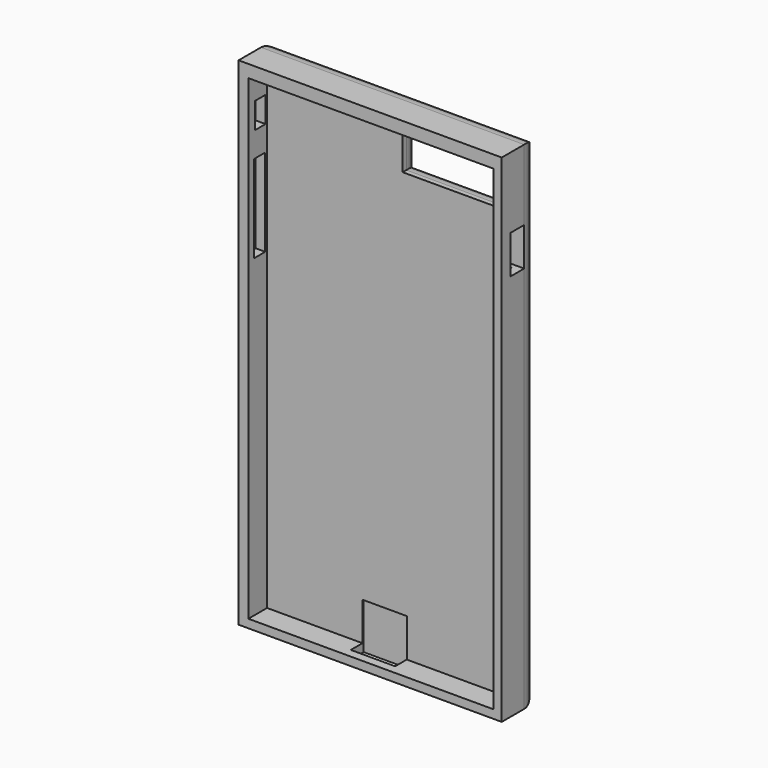
from build123d import *

# Parameters (mm, degrees)
F0_W          = 71.5089328587
F0_H          = 135.0168734789
F1_DEPTH      = 12.7
F2_W          = 66.5551535785
F2_H          = 129.3334215879
F3_DEPTH      = 3.175
F4_W          = 29.7537194565
F4_H          = 13.0016170442
F5_DEPTH      = 12.7
F6_T1_DEPTH   = 96.9089328587
F6_T3_DEPTH   = 160.4168734789
F6_T5_DEPTH   = 13.0016170442
F6_T7_DEPTH   = 29.7537194565
F6_T13_DEPTH  = 25.7016170442
F6_T17_DEPTH  = 42.4537194565
F6_T24_DEPTH  = 25.7016170442
F6_T29_DEPTH  = 42.4537194565
F6_T37_DEPTH  = 42.4537194565
F6_T42_DEPTH  = 25.7016170442
F6_T50_DEPTH  = 25.7016170442
F6_T56_DEPTH  = 42.4537194565
F8_W          = 12.041549664
F8_H          = 4.3452125974
F9_DEPTH      = 12.7
F10_DEPTH     = 3.175
F11_W         = 4.6954765302
F11_H         = 10.42952016
F12_DEPTH     = 1.5875
F13_DEPTH     = 3.175
F14_DEPTH     = 3.175
F15_W         = 3.5004382953
F15_H         = 7.000874728
F16_DEPTH     = 6.35
F17_W         = 3.7472322583
F17_H         = 23.7555298954
F18_DEPTH     = 6.35
F19_TEXT_SIZE = 6.2507784201
F20_DEPTH     = 5.842
F21_TEXT_SIZE = 8.6816441682
F22_DEPTH     = 5.08


# Not quite as in the source:
# - a fillet or chamfer that OpenCascade refuses, or shapes differently, is made with other operations: its cross-section is extruded or revolved along the edge and cut away or added
# - Text() gives the source's letters only with a copy of the font that has no kerning and outlines rounded to 1/6400 em; it was checked with that copy


with BuildPart() as f1:
    # F0 (on Front) → F1 (new body)
    with BuildSketch(Plane.XZ):
        with Locations((-0.6250794977, -1.1251419783)):
            Rectangle(F0_W, F0_H)
    extrude(amount=F1_DEPTH)

    # F2 (on face) → F3 (cut)
    with BuildSketch(Plane.XZ.offset(12.7)):
        with Locations((-0.4404280335, -1.6757398844)):
            Rectangle(F2_W, F2_H)
    extrude(amount=-F3_DEPTH, mode=Mode.SUBTRACT)

    # F4 (on face) → F5 (cut)
    with BuildSketch(Plane(origin=(0, 0, 0), x_dir=(-1, 0, 0), z_dir=(0, 1, 0))):
        with Locations((-18.0022506975, 56.3820470124)):
            Rectangle(F4_W, F4_H)
    extrude(amount=-F5_DEPTH, mode=Mode.SUBTRACT)

    # F6: fillet of radius 5.08 on 8 edges, made by hand

    # F6_s2 → F6_t1 (cut)
    with BuildSketch(Plane.YZ.offset(-49.079545927)):
        with BuildLine():
            ThreePointArc((-5.08, 66.3832947612), (-1.4878975516, 64.8953972096), (0, 61.3032947612))
            Line((0, 61.3032947612), (0, 66.3832947612))
            Line((0, 66.3832947612), (-5.08, 66.3832947612))
        make_face()
        with BuildLine():
            ThreePointArc((0, -63.5535787177), (-1.4878975516, -67.1456811661), (-5.08, -68.6335787177))
            Line((-5.08, -68.6335787177), (0, -68.6335787177))
            Line((0, -68.6335787177), (0, -63.5535787177))
        make_face()
    extrude(amount=F6_T1_DEPTH, mode=Mode.SUBTRACT)

    # F6_s4 → F6_t3 (cut)
    with BuildSketch(Plane.XY.offset(-81.3335787177)):
        with BuildLine():
            ThreePointArc((35.1293869317, -5.08), (33.6414893801, -1.4878975516), (30.0493869317, 0))
            Line((30.0493869317, 0), (35.1293869317, 0))
            Line((35.1293869317, 0), (35.1293869317, -5.08))
        make_face()
        with BuildLine():
            ThreePointArc((-36.379545927, -5.08), (-34.8916483755, -1.4878975516), (-31.299545927, 0))
            Line((-31.299545927, 0), (-36.379545927, 0))
            Line((-36.379545927, 0), (-36.379545927, -5.08))
        make_face()
    extrude(amount=F6_T3_DEPTH, mode=Mode.SUBTRACT)

    # F6_s6 → F6_t5 (cut)
    with BuildSketch(Plane.XY.offset(49.8812384903)):
        with BuildLine():
            ThreePointArc((-1.9546090308, 0), (1.6374934176, -1.4878975516), (3.1253909692, -5.08))
            Line((3.1253909692, -5.08), (3.1253909692, 0))
            Line((3.1253909692, 0), (-1.9546090308, 0))
        make_face()
        with BuildLine():
            ThreePointArc((37.9591104257, 0), (34.3670079773, -1.4878975516), (32.8791104257, -5.08))
            Line((32.8791104257, -5.08), (32.8791104257, 0))
            Line((32.8791104257, 0), (37.9591104257, 0))
        make_face()
    extrude(amount=F6_T5_DEPTH, mode=Mode.SUBTRACT)

    # F6_s8 → F6_t7 (cut)
    with BuildSketch(Plane.YZ.offset(3.1253909692)):
        with BuildLine():
            ThreePointArc((0, 44.8012384903), (-1.4878975516, 48.3933409388), (-5.08, 49.8812384903))
            Line((-5.08, 49.8812384903), (0, 49.8812384903))
            Line((0, 49.8812384903), (0, 44.8012384903))
        make_face()
        with BuildLine():
            ThreePointArc((0, 67.9628555346), (-1.4878975516, 64.3707530861), (-5.08, 62.8828555346))
            Line((-5.08, 62.8828555346), (0, 62.8828555346))
            Line((0, 62.8828555346), (0, 67.9628555346))
        make_face()
    extrude(amount=F6_T7_DEPTH, mode=Mode.SUBTRACT)


with BuildPart() as f6_tool11:
    # F6_s12 → F6_t13 (new body)
    with BuildSketch(Plane.XY.offset(37.1812384903)):
        with BuildLine():
            ThreePointArc((-1.9546090308, 0), (1.6374934176, -1.4878975516), (3.1253909692, -5.08))
            Line((3.1253909692, -5.08), (3.1253909692, 0))
            Line((3.1253909692, 0), (-1.9546090308, 0))
        make_face()
    extrude(amount=F6_T13_DEPTH)

    split(bisect_by=Plane.XY.offset(49.8812384903), keep=Keep.BOTTOM)


with BuildPart() as f6_tool15:
    # F6_s16 → F6_t17 (new body)
    with BuildSketch(Plane.YZ.offset(32.8791104257)):
        with BuildLine():
            ThreePointArc((0, 44.8012384903), (-1.4878975516, 48.3933409388), (-5.08, 49.8812384903))
            Line((-5.08, 49.8812384903), (0, 49.8812384903))
            Line((0, 49.8812384903), (0, 44.8012384903))
        make_face()
    extrude(amount=-F6_T17_DEPTH)

    split(bisect_by=Plane.YZ.offset(3.1253909692), keep=Keep.BOTTOM)


with BuildPart() as f6_tool11_1:
    add(f6_tool11.part)

    # F6_t19: intersect F6_tool15
    add(f6_tool15.part, mode=Mode.INTERSECT)


with BuildPart() as f1_1:
    add(f1.part)

    # F6_t9: cut F6_tool11
    add(f6_tool11_1.part, mode=Mode.SUBTRACT)


with BuildPart() as f6_tool22:
    # F6_s23 → F6_t24 (new body)
    with BuildSketch(Plane.XY.offset(49.8812384903)):
        with BuildLine():
            ThreePointArc((-1.9546090308, 0), (1.6374934176, -1.4878975516), (3.1253909692, -5.08))
            Line((3.1253909692, -5.08), (3.1253909692, 0))
            Line((3.1253909692, 0), (-1.9546090308, 0))
        make_face()
    extrude(amount=F6_T24_DEPTH)

    split(bisect_by=Plane.XY.offset(66.3832947612), keep=Keep.BOTTOM)

    split(bisect_by=Plane.XY.offset(62.8828555346), keep=Keep.TOP)


with BuildPart() as f6_tool27:
    # F6_s28 → F6_t29 (new body)
    with BuildSketch(Plane.YZ.offset(-9.5746090308)):
        with BuildLine():
            ThreePointArc((0, 67.9628555346), (-1.4878975516, 64.3707530861), (-5.08, 62.8828555346))
            Line((-5.08, 62.8828555346), (0, 62.8828555346))
            Line((0, 62.8828555346), (0, 67.9628555346))
        make_face()
    extrude(amount=F6_T29_DEPTH)

    split(bisect_by=Plane.XY.offset(66.3832947612), keep=Keep.BOTTOM)

    split(bisect_by=Plane.YZ.offset(3.1253909692), keep=Keep.BOTTOM)


with BuildPart() as f6_tool22_1:
    add(f6_tool22.part)

    # F6_t32: intersect F6_tool27
    add(f6_tool27.part, mode=Mode.INTERSECT)


with BuildPart() as f1_2:
    add(f1_1.part)

    # F6_t20: cut F6_tool22
    add(f6_tool22_1.part, mode=Mode.SUBTRACT)


with BuildPart() as f6_tool35:
    # F6_s36 → F6_t37 (new body)
    with BuildSketch(Plane.YZ.offset(45.5791104257)):
        with BuildLine():
            ThreePointArc((0, 44.8012384903), (-1.4878975516, 48.3933409388), (-5.08, 49.8812384903))
            Line((-5.08, 49.8812384903), (0, 49.8812384903))
            Line((0, 49.8812384903), (0, 44.8012384903))
        make_face()
    extrude(amount=-F6_T37_DEPTH)

    split(bisect_by=Plane.YZ.offset(35.1293869317), keep=Keep.BOTTOM)

    split(bisect_by=Plane.YZ.offset(32.8791104257), keep=Keep.TOP)


with BuildPart() as f6_tool40:
    # F6_s41 → F6_t42 (new body)
    with BuildSketch(Plane.XY.offset(62.8828555346)):
        with BuildLine():
            ThreePointArc((37.9591104257, 0), (34.3670079773, -1.4878975516), (32.8791104257, -5.08))
            Line((32.8791104257, -5.08), (32.8791104257, 0))
            Line((32.8791104257, 0), (37.9591104257, 0))
        make_face()
    extrude(amount=-F6_T42_DEPTH)

    split(bisect_by=Plane.YZ.offset(35.1293869317), keep=Keep.BOTTOM)

    split(bisect_by=Plane.XY.offset(49.8812384903), keep=Keep.BOTTOM)


with BuildPart() as f6_tool35_1:
    add(f6_tool35.part)

    # F6_t45: intersect F6_tool40
    add(f6_tool40.part, mode=Mode.INTERSECT)


with BuildPart() as f1_3:
    add(f1_2.part)

    # F6_t33: cut F6_tool35
    add(f6_tool35_1.part, mode=Mode.SUBTRACT)


with BuildPart() as f6_tool48:
    # F6_s49 → F6_t50 (new body)
    with BuildSketch(Plane.XY.offset(75.5828555346)):
        with BuildLine():
            ThreePointArc((37.9591104257, 0), (34.3670079773, -1.4878975516), (32.8791104257, -5.08))
            Line((32.8791104257, -5.08), (32.8791104257, 0))
            Line((32.8791104257, 0), (37.9591104257, 0))
        make_face()
    extrude(amount=-F6_T50_DEPTH)

    split(bisect_by=Plane.XY.offset(66.3832947612), keep=Keep.BOTTOM)

    split(bisect_by=Plane.YZ.offset(35.1293869317), keep=Keep.BOTTOM)

    split(bisect_by=Plane.XY.offset(62.8828555346), keep=Keep.TOP)


with BuildPart() as f6_tool54:
    # F6_s55 → F6_t56 (new body)
    with BuildSketch(Plane.YZ.offset(3.1253909692)):
        with BuildLine():
            ThreePointArc((0, 67.9628555346), (-1.4878975516, 64.3707530861), (-5.08, 62.8828555346))
            Line((-5.08, 62.8828555346), (0, 62.8828555346))
            Line((0, 62.8828555346), (0, 67.9628555346))
        make_face()
    extrude(amount=F6_T56_DEPTH)

    split(bisect_by=Plane.XY.offset(66.3832947612), keep=Keep.BOTTOM)

    split(bisect_by=Plane.YZ.offset(35.1293869317), keep=Keep.BOTTOM)

    split(bisect_by=Plane.YZ.offset(32.8791104257), keep=Keep.TOP)


with BuildPart() as f6_tool48_1:
    add(f6_tool48.part)

    # F6_t60: intersect F6_tool54
    add(f6_tool54.part, mode=Mode.INTERSECT)


with BuildPart() as f1_4:
    add(f1_3.part)

    # F6_t46: cut F6_tool48
    add(f6_tool48_1.part, mode=Mode.SUBTRACT)

    # F8 (on face) → F9 (cut)
    with BuildSketch(Plane(origin=(0, 0, -68.6335787177), x_dir=(1, 0, 0), z_dir=(0, 0, -1))):
        with Locations((-1.775913639, 8.129889844)):
            Rectangle(F8_W, F8_H)
    extrude(amount=-F9_DEPTH, mode=Mode.SUBTRACT)

    # F10 (cut): a face of the model
    f10_faces = [f1_4.faces().sort_by_distance(p)[0] for p in [
        (-1.2987269052, -9.525, -3.5253605956),
    ]]
    extrude(f10_faces, amount=-F10_DEPTH, mode=Mode.SUBTRACT)

    # F11 (on face) → F12 (join)
    with BuildSketch(Plane.YZ.offset(35.1293869317)):
        with Locations((-7.4277382651, 41.9391449541)):
            Rectangle(F11_W, F11_H)
    extrude(amount=F12_DEPTH)

    # F13 (cut): a face of the model
    f13_faces = [f1_4.faces().sort_by_distance(p)[0] for p in [
        (36.7168869317, -7.4277382651, 41.9391449541),
    ]]
    extrude(f13_faces, amount=-F13_DEPTH, mode=Mode.SUBTRACT)

    # F14 (cut): a face of the model
    f14_faces = [f1_4.faces().sort_by_distance(p)[0] for p in [
        (33.5418869317, -7.4277382651, 41.9391449541),
    ]]
    extrude(f14_faces, amount=-F14_DEPTH, mode=Mode.SUBTRACT)

    # F15 (on face) → F16 (cut)
    with BuildSketch(Plane(origin=(-36.379545927, 0, 0), x_dir=(0, -1, 0), z_dir=(-1, 0, 0))):
        with Locations((8.6260777898, 53.1316418201)):
            Rectangle(F15_W, F15_H)
    extrude(amount=-F16_DEPTH, mode=Mode.SUBTRACT)

    # F17 (on face) → F18 (cut)
    with BuildSketch(Plane(origin=(-36.379545927, 0, 0), x_dir=(0, -1, 0), z_dir=(-1, 0, 0))):
        with Locations((8.8518634439, 30.9905847535)):
            Rectangle(F17_W, F17_H)
    extrude(amount=-F18_DEPTH, mode=Mode.SUBTRACT)

    # F19 (on face) → F20 (join)
    with BuildSketch(Plane(origin=(0, 0, 0), x_dir=(-1, 0, 0), z_dir=(0, 1, 0))):
        with Locations((-18.8773591071, -49.6261417866)):
            Text('Palm Tree', F19_TEXT_SIZE, font='Open Sans', text_align=(TextAlign.LEFT, TextAlign.BOTTOM))
        with Locations((-18.8773591071, -58.1272004379)):
            Text('Phone Cases', F19_TEXT_SIZE, font='Open Sans', text_align=(TextAlign.LEFT, TextAlign.BOTTOM))
    extrude(amount=-F20_DEPTH)

    # F21 (on face) → F22 (cut)
    with BuildSketch(Plane(origin=(0, 0, 0), x_dir=(-1, 0, 0), z_dir=(0, 1, 0))):
        with Locations((-24.3780473247, -44.6305759251)):
            Text('Palm Tree', F21_TEXT_SIZE, font='Open Sans', text_align=(TextAlign.LEFT, TextAlign.BOTTOM))
        with Locations((-24.3780473247, -56.4376119938)):
            Text('Phone Cases', F21_TEXT_SIZE, font='Open Sans', text_align=(TextAlign.LEFT, TextAlign.BOTTOM))
    extrude(amount=-F22_DEPTH, mode=Mode.SUBTRACT)


solid = f1_4.part
